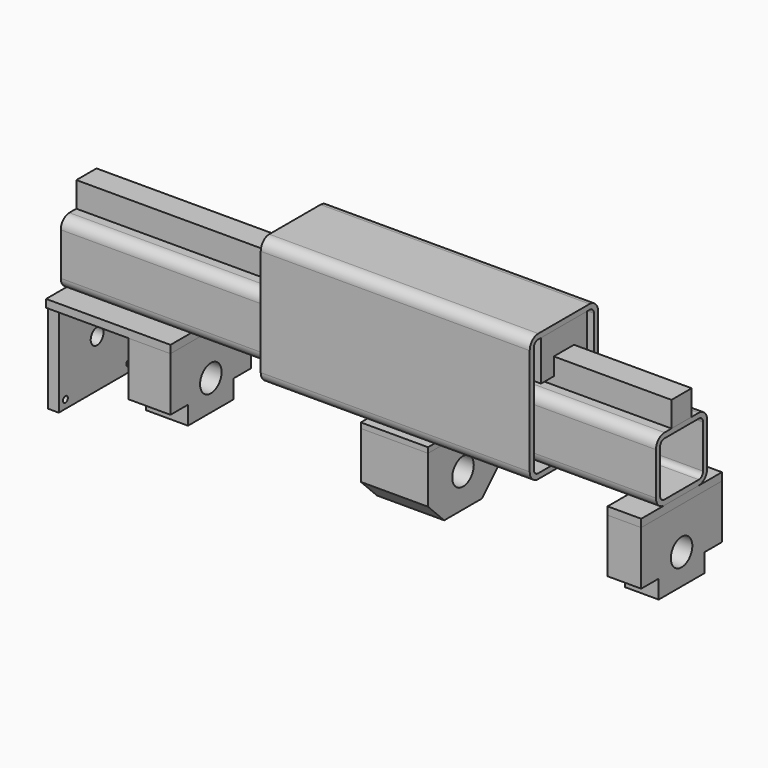
from build123d import *

# Parameters (mm, degrees)
F5_R      = 1.7859375
F5_R_2    = 4.7625
F7_DEPTH  = 6.35
F8_START  = 49
F4_R      = 8
F8_DEPTH  = 25
F9_START  = 124
F9_DEPTH  = 160
F10_DEPTH = 354
F11_START = 184
F0_R      = 8
F11_DEPTH = 40
F4_W      = 60
F4_H      = 4.6269972401
F12_DEPTH = 74
F13_START = 334
F13_DEPTH = 20
F14_START = 334
F14_DEPTH = 20
F15_START = 184
F15_DEPTH = 40
F2_W      = 15
F2_H      = 10.4
F2_H_2    = 4.6
F16_DEPTH = 354
F17_START = 124
F17_DEPTH = 60
F18_START = 224
F18_DEPTH = 60


# Not quite as in the source:
# - ends of sketch curves that miss each other by under 0.0002 mm in the source are joined


with BuildPart() as f7:
    # F5 (on Right) → F7 (new body, through all)
    with BuildSketch(Plane.YZ):
        with BuildLine():
            ThreePointArc((-22.5073760265, 25.0000027599), (-21.9607180856, 24.3647120661), (-21.7640625, 23.55))
            ThreePointArc((-21.7640625, 23.55), (-24.3647120661, 21.9607180856), (-24.5926239735, 25.0000027599))
            Line((-24.5926239735, 25.0000027599), (-28.5, 25.0000027599))
            Line((-28.5, 25.0000027599), (-28.5, -28.5))
            Line((-28.5, -28.5), (28.5, -28.5))
            Line((28.5, -28.5), (28.5, 25.0000027599))
            Line((28.5, 25.0000027599), (24.5926239735, 25.0000027599))
            ThreePointArc((24.5926239735, 25.0000027599), (25.1392819144, 24.3647120661), (25.3359375, 23.55))
            ThreePointArc((25.3359375, 23.55), (22.7352879339, 21.9607180856), (22.5073760265, 25.0000027599))
            Line((22.5073760265, 25.0000027599), (-22.5073760265, 25.0000027599))
        make_face()
        with Locations((-23.55, -23.55)):
            Circle(F5_R, mode=Mode.SUBTRACT)
        with Locations((23.55, -23.55)):
            Circle(F5_R, mode=Mode.SUBTRACT)
        Circle(F5_R_2, mode=Mode.SUBTRACT)
    extrude(amount=F7_DEPTH)


with BuildPart() as f8:
    # F4 (on Right) → F8 (new body)
    with BuildSketch(Plane.YZ.offset(F8_START)):
        Polygon((30, 25.0000027599), (-30, 24.9999972401), (-30, -7.0000027599), (-17, -7.0000027599), (-17, -18.0000027599), (17, -18.0000027599), (17, -7.0000027599), (30, -7.0000027599), align=None)
        Circle(F4_R, mode=Mode.SUBTRACT)
    extrude(amount=F8_DEPTH)


with BuildPart() as f9:
    # F1 (on Right) → F9 (new body)
    with BuildSketch(Plane.YZ.offset(F9_START)):
        with BuildLine():
            ThreePointArc((25.4, 93.025), (23.5401280605, 97.5151280605), (19.05, 99.375))
            Line((19.05, 99.375), (-19.05, 99.375))
            ThreePointArc((-19.05, 99.375), (-23.5401280605, 97.5151280605), (-25.4, 93.025))
            Line((-25.4, 93.025), (-25.4, 29.525))
            ThreePointArc((-25.4, 29.525), (-23.5401280605, 25.0348719395), (-19.05, 23.175))
            Line((-19.05, 23.175), (19.05, 23.175))
            ThreePointArc((19.05, 23.175), (23.5401280605, 25.0348719395), (25.4, 29.525))
            Line((25.4, 29.525), (25.4, 93.025))
        make_face()
        with BuildLine():
            Line((-19.177, 96.327), (19.177, 96.327))
            ThreePointArc((19.177, 96.327), (21.4220640303, 95.3970640303), (22.352, 93.152))
            Line((22.352, 93.152), (22.352, 29.398))
            ThreePointArc((22.352, 29.398), (21.4220640303, 27.1529359697), (19.177, 26.223))
            Line((19.177, 26.223), (-19.177, 26.223))
            ThreePointArc((-19.177, 26.223), (-21.4220640303, 27.1529359697), (-22.352, 29.398))
            Line((-22.352, 29.398), (-22.352, 93.152))
            ThreePointArc((-22.352, 93.152), (-21.4220640303, 95.3970640303), (-19.177, 96.327))
        make_face(mode=Mode.SUBTRACT)
    extrude(amount=F9_DEPTH)


with BuildPart() as f10:
    # F3 (on Right) → F10 (new body, through all)
    with BuildSketch(Plane.YZ):
        with BuildLine():
            ThreePointArc((19.05, 61.377), (17.1901280605, 65.8671280605), (12.7, 67.727))
            Line((12.7, 67.727), (-12.7, 67.727))
            ThreePointArc((-12.7, 67.727), (-17.1901280605, 65.8671280605), (-19.05, 61.377))
            Line((-19.05, 61.377), (-19.05, 35.977))
            ThreePointArc((-19.05, 35.977), (-17.1901280605, 31.4868719395), (-12.7, 29.627))
            Line((-12.7, 29.627), (12.7, 29.627))
            ThreePointArc((12.7, 29.627), (17.1901280605, 31.4868719395), (19.05, 35.977))
            Line((19.05, 35.977), (19.05, 61.377))
        make_face()
        with BuildLine():
            Line((-12.827, 64.679), (12.827, 64.679))
            ThreePointArc((12.827, 64.679), (15.0720640303, 63.7490640303), (16.002, 61.504))
            Line((16.002, 61.504), (16.002, 35.85))
            ThreePointArc((16.002, 35.85), (15.0720640303, 33.6049359697), (12.827, 32.675))
            Line((12.827, 32.675), (-12.827, 32.675))
            ThreePointArc((-12.827, 32.675), (-15.0720640303, 33.6049359697), (-16.002, 35.85))
            Line((-16.002, 35.85), (-16.002, 61.504))
            ThreePointArc((-16.002, 61.504), (-15.0720640303, 63.7490640303), (-12.827, 64.679))
        make_face(mode=Mode.SUBTRACT)
    extrude(amount=F10_DEPTH)


with BuildPart() as f11:
    # F0 (on Right) → F11 (new body)
    with BuildSketch(Plane.YZ.offset(F11_START)):
        Polygon((26, 20), (-26, 20), (-26, -7.9791847198), (-13.9791847198, -20), (13.9791847198, -20), (26, -7.9791847198), align=None)
        Circle(F0_R, mode=Mode.SUBTRACT)
    extrude(amount=F11_DEPTH)


with BuildPart() as f12:
    # F4 (on Right) → F12 (new body, through all)
    with BuildSketch(Plane.YZ):
        with Locations((0, 27.31350138)):
            Rectangle(F4_W, F4_H)
    extrude(amount=F12_DEPTH)


with BuildPart() as f13:
    # F4 (on Right) → F13 (new body)
    with BuildSketch(Plane.YZ.offset(F13_START)):
        Polygon((30, 25.0000027599), (-30, 24.9999972401), (-30, -7.0000027599), (-17, -7.0000027599), (-17, -18.0000027599), (17, -18.0000027599), (17, -7.0000027599), (30, -7.0000027599), align=None)
        Circle(F4_R, mode=Mode.SUBTRACT)
    extrude(amount=F13_DEPTH)


with BuildPart() as f14:
    # F4 (on Right) → F14 (new body)
    with BuildSketch(Plane.YZ.offset(F14_START)):
        with Locations((0, 27.31350138)):
            Rectangle(F4_W, F4_H)
    extrude(amount=F14_DEPTH)


with BuildPart() as f15:
    # F1 (on Right) → F15 (new body)
    with BuildSketch(Plane.YZ.offset(F15_START)):
        Polygon((26, 23.175), (19.05, 23.175), (-19.05, 23.175), (-26, 23.175), (-26, 20), (26, 20), align=None)
    extrude(amount=F15_DEPTH)


with BuildPart() as f16:
    # F2 (on Right) → F16 (new body, through all)
    with BuildSketch(Plane.YZ):
        with Locations((0, 77.527)):
            Rectangle(F2_W, F2_H)
        with Locations((0, 70.027)):
            Rectangle(F2_W, F2_H_2)
    extrude(amount=F16_DEPTH)


with BuildPart() as f17:
    # F2 (on Right) → F17 (new body)
    with BuildSketch(Plane.YZ.offset(F17_START)):
        Polygon((7.5, 82.727), (7.5, 72.327), (17, 72.327), (17, 96.327), (-17, 96.327), (-17, 72.327), (-7.5, 72.327), (-7.5, 82.727), align=None)
    extrude(amount=F17_DEPTH)


with BuildPart() as f18:
    # F2 (on Right) → F18 (new body)
    with BuildSketch(Plane.YZ.offset(F18_START)):
        Polygon((7.5, 82.727), (7.5, 72.327), (17, 72.327), (17, 96.327), (-17, 96.327), (-17, 72.327), (-7.5, 72.327), (-7.5, 82.727), align=None)
    extrude(amount=F18_DEPTH)


solid = Compound([f7.part, f8.part, f9.part, f10.part, f11.part, f12.part, f13.part, f14.part, f15.part, f16.part, f17.part, f18.part])
